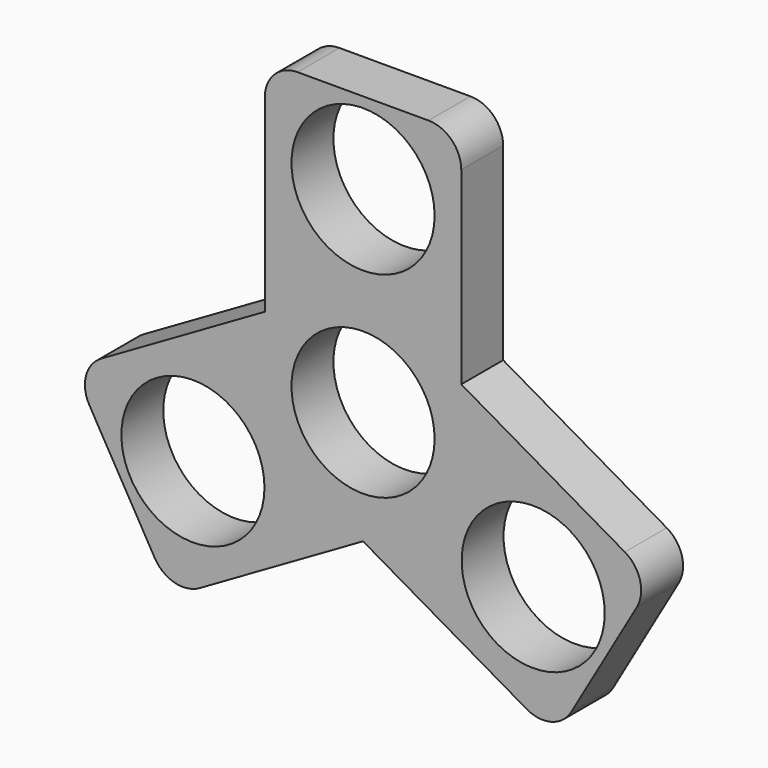
from build123d import *

# Parameters (mm, degrees)
F0_R     = 10.925
F1_DEPTH = 8


with BuildPart() as f1:
    # F0 (on Front) → F1 (new body)
    with BuildSketch(Plane.XZ):
        with BuildLine():
            ThreePointArc((227.1570374133, 320.1293041687), (225.6925713192, 323.6648380746), (222.1570374133, 325.1293041687))
            Line((222.1570374133, 325.1293041687), (202.1570374133, 325.1293041687))
            ThreePointArc((202.1570374133, 325.1293041687), (198.6215035074, 323.6648380746), (197.1570374133, 320.1293041687))
            Line((197.1570374133, 320.1293041687), (197.1570374133, 291.2895582065))
            Line((197.1570374133, 291.2895582065), (205.5064023187, 296.1100662822))
            Line((205.5064023187, 296.1100662822), (208.831719866, 301.8696852254))
            Line((208.831719866, 301.8696852254), (212.1570374133, 299.9498122444))
            Line((212.1570374133, 299.9498122444), (215.4823549606, 301.8696852254))
            Line((215.4823549606, 301.8696852254), (218.8076725079, 296.1100662822))
            Line((218.8076725079, 296.1100662822), (227.1570374133, 291.2895582065))
            Line((227.1570374133, 291.2895582065), (227.1570374133, 320.1293041687))
        make_face()
        with Locations((212.1570374133, 312.6293041687)):
            Circle(F0_R, mode=Mode.SUBTRACT)
        with BuildLine():
            Line((252.1329900552, 276.8696852254), (227.1570374133, 291.2895582065))
            Line((227.1570374133, 291.2895582065), (227.1570374133, 281.6485420551))
            Line((227.1570374133, 281.6485420551), (230.4823549606, 275.8889231119))
            Line((230.4823549606, 275.8889231119), (227.1570374133, 273.9690501308))
            Line((227.1570374133, 273.9690501308), (227.1570374133, 270.1293041687))
            Line((227.1570374133, 270.1293041687), (220.5064023187, 270.1293041687))
            Line((220.5064023187, 270.1293041687), (212.1570374133, 265.308796093))
            Line((212.1570374133, 265.308796093), (237.1329900552, 250.8889231119))
            ThreePointArc((237.1329900552, 250.8889231119), (240.9270852807, 250.3894209994), (243.9631170741, 252.7190501308))
            Line((243.9631170741, 252.7190501308), (253.9631170741, 270.0395582065))
            ThreePointArc((253.9631170741, 270.0395582065), (254.4626191867, 273.833653432), (252.1329900552, 276.8696852254))
        make_face()
        with Locations((238.1377995268, 267.6293041687)):
            Circle(F0_R, mode=Mode.SUBTRACT)
        Polygon((227.1570374133, 281.6485420551), (227.1570374133, 291.2895582065), (218.8076725079, 296.1100662822), align=None)
        Polygon((205.5064023187, 296.1100662822), (197.1570374133, 291.2895582065), (197.1570374133, 281.6485420551), align=None)
        with BuildLine():
            Line((197.1570374133, 281.6485420551), (197.1570374133, 291.2895582065))
            Line((197.1570374133, 291.2895582065), (172.1810847714, 276.8696852254))
            ThreePointArc((172.1810847714, 276.8696852254), (169.8514556399, 273.833653432), (170.3509577525, 270.0395582065))
            Line((170.3509577525, 270.0395582065), (180.3509577525, 252.7190501308))
            ThreePointArc((180.3509577525, 252.7190501308), (183.3869895459, 250.3894209994), (187.1810847714, 250.8889231119))
            Line((187.1810847714, 250.8889231119), (212.1570374133, 265.308796093))
            Line((212.1570374133, 265.308796093), (203.8076725079, 270.1293041687))
            Line((203.8076725079, 270.1293041687), (197.1570374133, 270.1293041687))
            Line((197.1570374133, 270.1293041687), (197.1570374133, 273.9690501308))
            Line((197.1570374133, 273.9690501308), (193.831719866, 275.8889231119))
            Line((193.831719866, 275.8889231119), (197.1570374133, 281.6485420551))
        make_face()
        with Locations((186.1762752998, 267.6293041687)):
            Circle(F0_R, mode=Mode.SUBTRACT)
        Polygon((212.1570374133, 265.308796093), (220.5064023187, 270.1293041687), (203.8076725079, 270.1293041687), align=None)
        Polygon((208.831719866, 301.8696852254), (205.5064023187, 296.1100662822), (212.1570374133, 299.9498122444), align=None)
        Polygon((212.1570374133, 299.9498122444), (218.8076725079, 296.1100662822), (215.4823549606, 301.8696852254), align=None)
        Polygon((227.1570374133, 273.9690501308), (227.1570374133, 281.6485420551), (218.8076725079, 296.1100662822), (212.1570374133, 299.9498122444), (205.5064023187, 296.1100662822), (197.1570374133, 281.6485420551), (197.1570374133, 273.9690501308), (203.8076725079, 270.1293041687), (220.5064023187, 270.1293041687), align=None)
        with Locations((212.1570374133, 282.6293041687)):
            Circle(F0_R, mode=Mode.SUBTRACT)
        Polygon((197.1570374133, 273.9690501308), (197.1570374133, 281.6485420551), (193.831719866, 275.8889231119), align=None)
        Polygon((203.8076725079, 270.1293041687), (197.1570374133, 273.9690501308), (197.1570374133, 270.1293041687), align=None)
        Polygon((227.1570374133, 270.1293041687), (227.1570374133, 273.9690501308), (220.5064023187, 270.1293041687), align=None)
        Polygon((230.4823549606, 275.8889231119), (227.1570374133, 281.6485420551), (227.1570374133, 273.9690501308), align=None)
    extrude(amount=F1_DEPTH)


solid = f1.part
